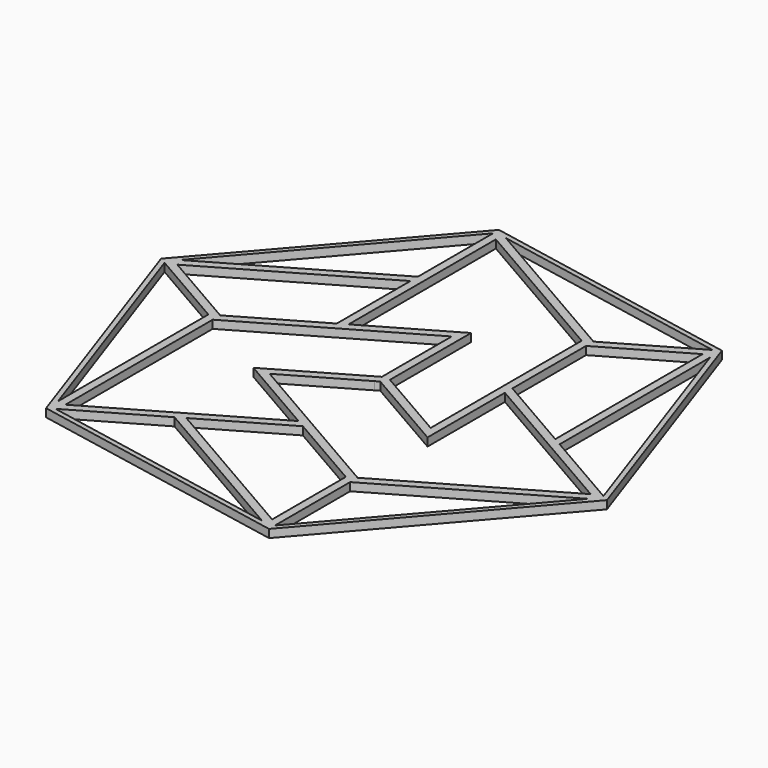
from build123d import *

# Parameters (mm, degrees)
F1_DEPTH = 2


# Not quite as in the source:
# - a feature names something its author has since deleted; it is built from what else it names


with BuildPart() as f1:
    # F0 (on Top) → F1 (new body)
    with BuildSketch(Plane.XY):
        Polygon((63.5912331811, -12.2381385313), (63.3644544975, -11.5834848612), (43.3012701892, 0), (43.3012701892, 46.333939444), (42.3941554539, 48.9525541272), (41.7138194028, 49.0834848613), (21.6506350946, 37.5000000002), (-18.4757335211, 60.6669697221), (-21.1970777272, 61.1906926587), (-21.6506350946, 60.6669697224), (-21.6506350946, 37.5), (-61.7770037106, 14.333030278), (-63.591233181, 12.2381385317), (-63.3644544972, 11.583484861), (-43.3012701894, 1e-10), (-43.3012701894, -46.3339394428), (-42.3941554538, -48.9525541268), (-41.7138194016, -49.0834848611), (-21.6506350939, -37.5000000002), (18.4757335209, -60.6669697216), (21.1970777272, -61.1906926583), (21.6506350946, -60.666969722), (21.6506350946, -37.5), (61.7770037099, -14.3330302784), align=None)
        Polygon((19.6506350946, -36.3452994616), (19.6506350946, -59.0358983857), (-19.6506350948, -36.3452994623), (5e-10, -25.0000000003), align=None, mode=Mode.SUBTRACT)
        Polygon((-1.0000000004, 0.5773502687), (-1.9999999999, -2e-10), (-22.6506350946, -11.9226497308), (-1.9999999997, -23.8452994618), (-41.3012701889, -46.535898385), (-41.3012701889, -1.1547005386), (-1.0000000004, 22.1132486534), (-1.0000000004, 1.7320508071), align=None, mode=Mode.SUBTRACT)
        Polygon((21.6506350946, 10.1905989232), (60.9519052838, -12.5), (21.6506350946, -35.1905989232), (-18.6506350946, -11.9226497308), (-1, -1.7320508076), (0, -1.1547005384), (21.6506350946, -13.6547005384), align=None, mode=Mode.SUBTRACT)
        Polygon((-60.9519052838, 12.5), (-21.6506350946, 35.1905989232), (-21.6506350946, 12.5000000002), (-41.3012701894, 1.1547005385), align=None, mode=Mode.SUBTRACT)
        Polygon((19.6506350946, -10.1905989242), (2, -1e-09), (1.0000000005, 0.5773502699), (1.0000000005, 1.7320508081), (1.0000000005, 25.5773502697), (-19.6506350952, 13.6547005382), (-19.6506350952, 59.0358983854), (19.6506350946, 36.3452994618), align=None, mode=Mode.SUBTRACT)
        Polygon((21.6506350946, 35.1905989229), (41.3012701896, 46.5358983847), (41.3012701896, 1.1547005382), (21.6506350946, 12.5), align=None, mode=Mode.SUBTRACT)
        Polygon((-21.6506350946, 60.6669697224), (-21.6506350946, 62.5000000002), (-64.9519052838, 12.5), (-61.7770037106, 14.333030278), align=None)
        Polygon((41.7138194028, 49.0834848613), (43.3012701892, 50.0000000002), (-21.6506350948, 62.5000000001), (-18.4757335211, 60.6669697221), align=None)
        Polygon((-64.9519052838, 12.5), (-43.301270189, -50), (-43.3012701894, -46.3339394428), (-63.3644544972, 11.583484861), align=None)
        Polygon((-61.7770037106, 14.333030278), (-64.9519052838, 12.5), (-63.3644544972, 11.583484861), (-63.591233181, 12.2381385317), align=None)
        Polygon((-43.3012701894, -46.3339394428), (-43.3012701894, -50.0000000007), (-41.7138194016, -49.0834848611), (-42.3941554538, -48.9525541268), align=None)
        Polygon((-43.301270189, -50), (21.6506350949, -62.4999999997), (18.4757335209, -60.6669697216), (-41.7138194016, -49.0834848611), align=None)
        Polygon((18.4757335209, -60.6669697216), (21.6506350946, -62.4999999998), (21.6506350946, -60.666969722), (21.1970777272, -61.1906926583), align=None)
        Polygon((21.6506350949, -62.4999999997), (64.9519052839, -12.4999999995), (61.7770037099, -14.3330302784), (21.6506350946, -60.666969722), align=None)
        Polygon((61.7770037099, -14.3330302784), (64.9519052838, -12.5), (63.3644544975, -11.5834848612), (63.5912331811, -12.2381385313), align=None)
        Polygon((63.3644544975, -11.5834848612), (64.9519052838, -12.5), (43.3012701891, 50.0000000004), (43.3012701892, 46.333939444), align=None)
        Polygon((43.3012701892, 46.333939444), (43.3012701892, 50.0000000002), (41.7138194028, 49.0834848613), (42.3941554539, 48.9525541272), align=None)
        Polygon((-18.4757335211, 60.6669697221), (-21.6506350946, 62.5000000002), (-21.6506350946, 60.6669697224), (-21.1970777272, 61.1906926587), align=None)
    extrude(amount=F1_DEPTH)


solid = f1.part
